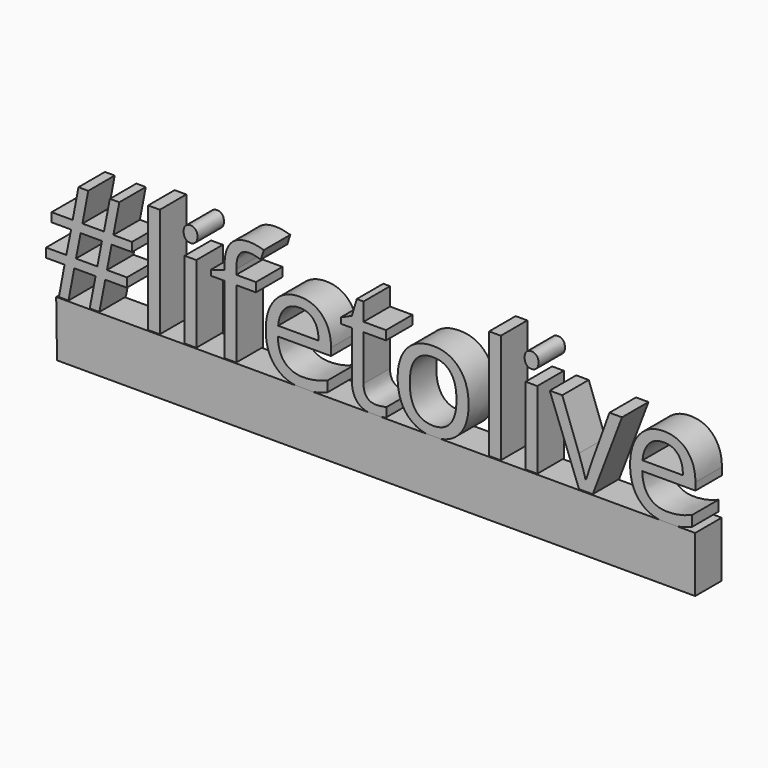
from build123d import *

# Parameters (mm, degrees)
F0_TEXT_SIZE = 33.2071360479
F1_DEPTH     = 7.62
F3_DEPTH     = 7.62


# Not quite as in the source:
# - Text() gives the source's letters only with a copy of the font that has no kerning and outlines rounded to 1/6400 em; it was checked with that copy


with BuildPart() as f1:
    # F0 (on Front) → F1 (new body)
    with BuildSketch(Plane.XZ):
        with Locations((-77.773033826, -13.5542016426)):
            Text('#lifetolive', F0_TEXT_SIZE, font='Open Sans', text_align=(TextAlign.LEFT, TextAlign.BOTTOM))
    extrude(amount=F1_DEPTH)


with BuildPart() as f3:
    # F2 (on Front) → F3 (new body)
    with BuildSketch(Plane.XZ):
        Polygon((72.4182873964, -13.7386163697), (-74.6218934655, -13.7386163697), (-74.4281560183, -26.5247188509), (72.4182873964, -26.5247188509), align=None)
    extrude(amount=F3_DEPTH)


solid = Compound([f1.part, f3.part])
